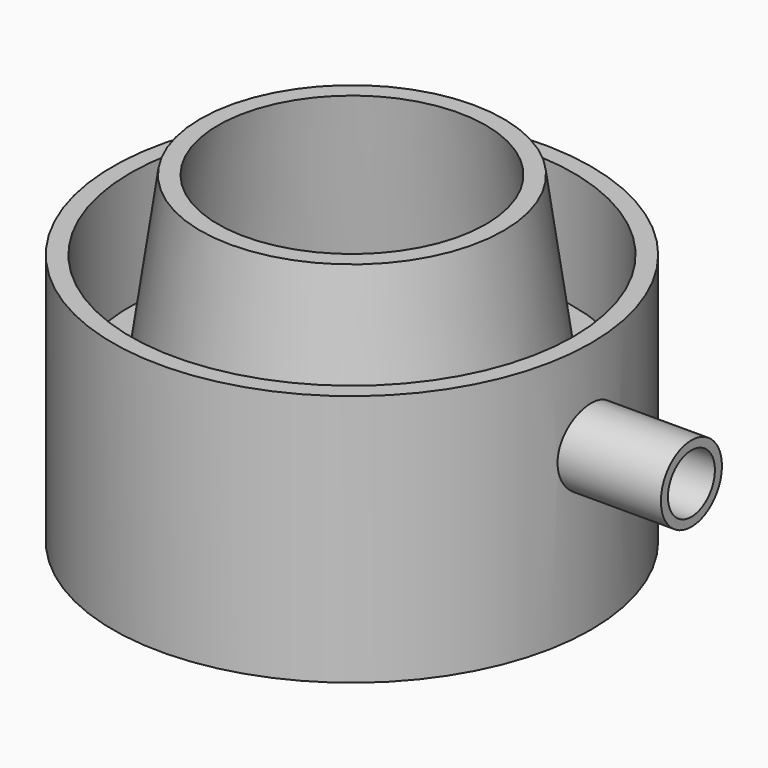
from build123d import *

# Parameters (mm, degrees)
F3_R     = 6.5
F3_R_2   = 5
F4_DEPTH = 20
F5_DEPTH = 14.3


with BuildPart() as f1:
    # F0 (on Front) → F1 (revolve)
    with BuildSketch(Plane.XZ):
        Polygon((-130.0127011951, 91.7292905117), (-133.0127011951, 91.7292905117), (-128.0937719805, 56.7292905117), (-118.0937719805, 56.7292905117), (-118.0937719805, 36.7292905117), (-115.0937719805, 36.7292905117), (-115.0937719805, 79.7292905117), (-118.0937719805, 79.7292905117), (-118.0937719805, 59.7292905117), (-125.5153944847, 59.7292905117), align=None)
    revolve(axis=Axis((-155.8437719805, 0, 54.1304184761), (0, 0, -1)))

    # F3 (on offset) → F4 (join)
    with BuildSketch(Plane.YZ.offset(-118)):
        with Locations((0, 64.2200395022)):
            Circle(F3_R)
        with Locations((0, 64.2200395022)):
            Circle(F3_R_2, mode=Mode.SUBTRACT)
    extrude(amount=F4_DEPTH)

    # F3 (on offset) → F5 (cut, symmetric)
    with BuildSketch(Plane.YZ.offset(-118)):
        with Locations((0, 64.2200395022)):
            Circle(F3_R_2)
    extrude(amount=F5_DEPTH, both=True, mode=Mode.SUBTRACT)


solid = f1.part
